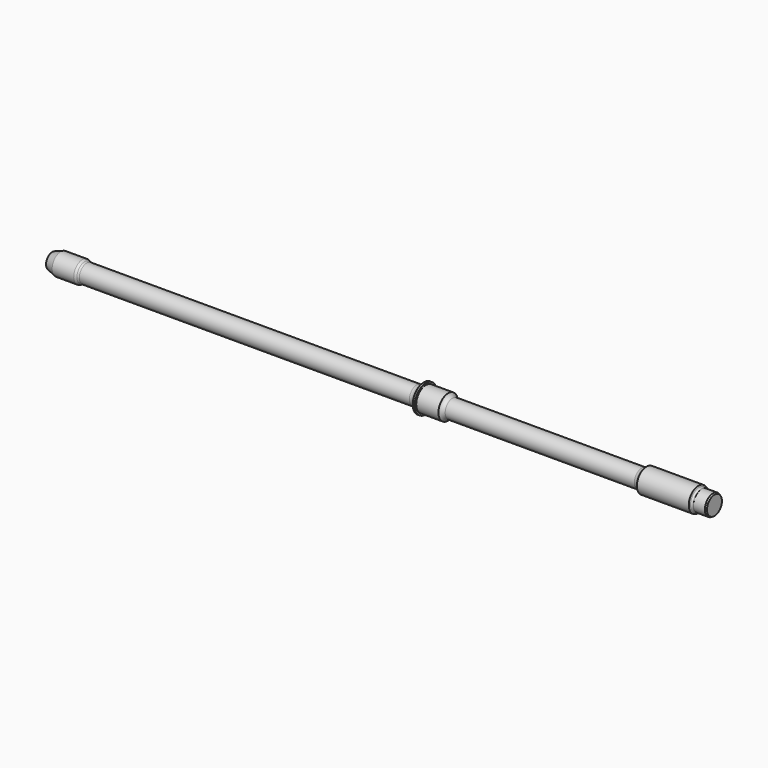
from build123d import *

# Parameters (mm, degrees)
F4_R = 0.25
F5_R = 5
F6_R = 5


# Not quite as in the source:
# - a fillet or chamfer that OpenCascade refuses, or shapes differently, is made with other operations: its cross-section is extruded or revolved along the edge and cut away or added


with BuildPart() as f1:
    # F0 (on Front) → F1 (revolve)
    with BuildSketch(Plane.XZ):
        with BuildLine():
            Line((-2, 9.525), (-350.6009565311, 9.525))
            Line((-350.6009565311, 9.525), (-354, 11.11))
            Line((-354, 11.11), (-376.25, 11.11))
            Line((-376.25, 11.11), (-385, 8))
            Line((-385, 8), (-385, 0))
            Line((-385, 0), (297.49, 0))
            Line((297.49, 0), (297.49, 9.6239745962))
            Line((297.49, 9.6239745962), (295.99, 10.49))
            Line((295.99, 10.49), (284.1809884429, 10.49))
            ThreePointArc((284.1809884429, 10.49), (282.8216403227, 10.297737003), (281.7297929543, 11.13))
            Line((281.7297929543, 11.13), (280.97, 12.446))
            Line((280.97, 12.446), (227.5, 12.446))
            Line((227.5, 12.446), (224.579, 9.525))
            Line((224.579, 9.525), (23, 9.525))
            Line((23, 9.525), (23, 12.495))
            Line((23, 12.495), (0, 12.495))
            Line((0, 12.495), (0, 14.35))
            Line((0, 14.35), (-2, 14.35))
            Line((-2, 14.35), (-2, 9.525))
        make_face()
    revolve(axis=Axis((-43.755, 0, 0), (-1, 0, 0)))

    # F2: fillet of radius 8 on 1 edges, made by hand

    # F2_s1 → F2_t2 (revolve)
    with BuildSketch(Plane.XZ):
        with BuildLine():
            ThreePointArc((-2, 14.35), (-4.9498048155, 10.8391941398), (-9.3429813428, 9.525))
            Line((-9.3429813428, 9.525), (-2, 9.525))
            Line((-2, 9.525), (-2, 14.35))
        make_face()
    revolve(axis=Axis((-2, 0, 0), (-1, 0, 0)))

    # F3: fillet of radius 5 on 1 edges, made by hand

    # F3_s1 → F3_t2 (revolve)
    with BuildSketch(Plane.XZ):
        with BuildLine():
            ThreePointArc((27.5693653826, 9.525), (24.8444800639, 10.3327452367), (23, 12.495))
            Line((23, 12.495), (23, 9.525))
            Line((23, 9.525), (27.5693653826, 9.525))
        make_face()
    revolve(axis=Axis((23, 0, 0), (-1, 0, 0)))

    # F4
    f4_edges = [f1.edges().sort_by_distance(p)[0] for p in [
        (0, 0, -12.495),
    ]]
    fillet(f4_edges, radius=F4_R)

    # F5
    f5_edges = [f1.edges().sort_by_distance(p)[0] for p in [
        (-350.600957, 0, -9.525),
    ]]
    fillet(f5_edges, radius=F5_R)

    # F6
    f6_edges = [f1.edges().sort_by_distance(p)[0] for p in [
        (224.579, 0, -9.525),
    ]]
    fillet(f6_edges, radius=F6_R)


solid = f1.part
